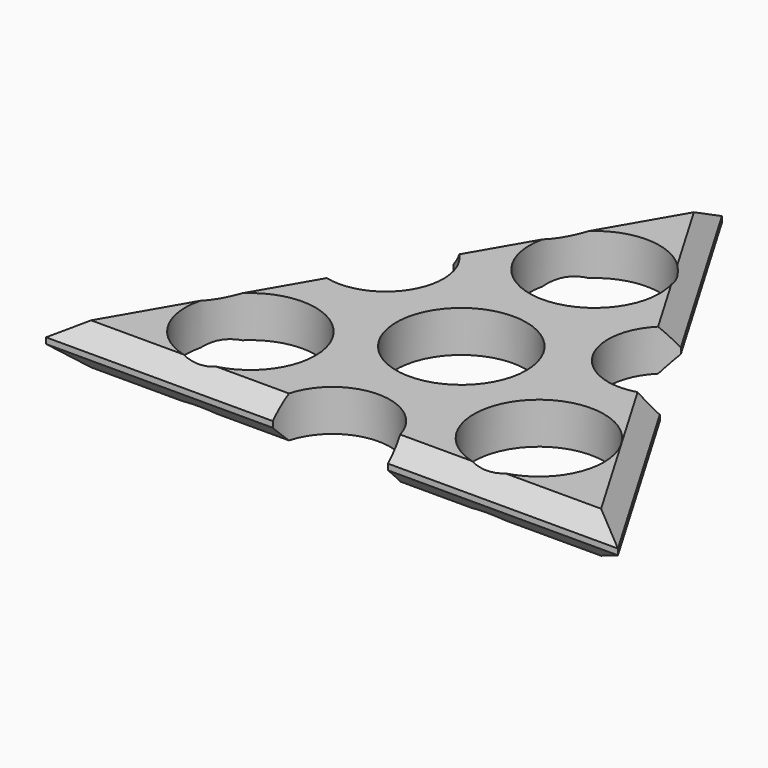
from build123d import *

# Parameters (mm, degrees)
F0_R         = 11
F1_DEPTH     = 7
F2_T1_DEPTH  = 53.4348218988
F2_T3_DEPTH  = 53.3566125342
F2_T5_DEPTH  = 53.6604130231
F2_T7_DEPTH  = 53.7564599562
F2_T9_DEPTH  = 54.3050348939
F2_T11_DEPTH = 54.0874720662
F3_T1_DEPTH  = 53.4348218988
F3_T3_DEPTH  = 53.6604130231
F3_T5_DEPTH  = 53.7564599562
F3_T7_DEPTH  = 54.3050348939
F3_T9_DEPTH  = 54.0874720662
F3_T11_DEPTH = 53.3566125342


# Not quite as in the source:
# - a fillet or chamfer that OpenCascade refuses, or shapes differently, is made with other operations: its cross-section is extruded or revolved along the edge and cut away or added


with BuildPart() as f1:
    # F0 (on Top) → F1 (new body)
    with BuildSketch(Plane.XY):
        with BuildLine():
            Line((19.2151323873, 22.3788071315), (0, 55.077418685))
            Line((0, 55.077418685), (-19.066227053, 22.2013174855))
            ThreePointArc((-19.066227053, 22.2013174855), (-15.2197508504, 8.7138440156), (-28.8366321548, 5.35410246))
            Line((-28.8366321548, 5.35410246), (-48.0160338648, -27.7171470225))
            Line((-48.0160338648, -27.7171470225), (-9.6896718364, -27.7171470225))
            ThreePointArc((-9.6896718364, -27.7171470225), (0.0445471902, -17.5375945189), (9.7787662169, -27.7171470225))
            Line((9.7787662169, -27.7171470225), (48.6537031829, -27.7171470225))
            Line((48.6537031829, -27.7171470225), (29.0682872932, 5.6115802214))
            ThreePointArc((29.0682872932, 5.6115802214), (15.2034219667, 8.7426653076), (19.2151323873, 22.3788071315))
        make_face()
        with Locations((-24.3902284877, -14.0817042541)):
            Circle(F0_R, mode=Mode.SUBTRACT)
        Circle(F0_R, mode=Mode.SUBTRACT)
        with Locations((24.3902285123, -14.0817042399)):
            Circle(F0_R, mode=Mode.SUBTRACT)
        with Locations((0, 28.1634107232)):
            Circle(F0_R, mode=Mode.SUBTRACT)
    extrude(amount=F1_DEPTH)

    # F2: chamfer of 3 on 6 edges, made by hand

    # F2_s2 → F2_t1 (cut)
    with BuildSketch(Plane(origin=(27.7729977796, 47.8892799857, 0), x_dir=(0, 0, 1), z_dir=(-0.5016804508, -0.8650530188, 0))):
        Polygon((4, 27.6312642329), (7, 24.6312642329), (7, 27.6312642329), align=None)
    extrude(amount=F2_T1_DEPTH, mode=Mode.SUBTRACT)

    # F2_s4 → F2_t3 (cut)
    with BuildSketch(Plane(origin=(-0.9341553956, 1.5896629696, 0), x_dir=(0, 0, 1), z_dir=(-0.5066411345, 0.8621570396, 0))):
        Polygon((4, 27.9044858871), (7, 24.9044858871), (7, 27.9044858871), align=None)
    extrude(amount=F2_T3_DEPTH, mode=Mode.SUBTRACT)

    # F2_s6 → F2_t5 (cut)
    with BuildSketch(Plane(origin=(-1.0636343753, -1.8340362392, 0), x_dir=(0, 0, 1), z_dir=(-0.5016804508, -0.8650530188, 0))):
        Polygon((4, 27.6312642329), (7, 24.6312642329), (7, 27.6312642329), align=None)
    extrude(amount=F2_T5_DEPTH, mode=Mode.SUBTRACT)

    # F2_s8 → F2_t7 (cut)
    with BuildSketch(Plane.YZ.offset(-55.7310828287)):
        Polygon((-27.7171470225, 4), (-24.7171470225, 7), (-27.7171470225, 7), align=None)
    extrude(amount=F2_T7_DEPTH, mode=Mode.SUBTRACT)

    # F2_s10 → F2_t9 (cut)
    with BuildSketch(Plane.YZ.offset(2.063717253)):
        Polygon((-27.7171470225, 4), (-24.7171470225, 7), (-27.7171470225, 7), align=None)
    extrude(amount=F2_T9_DEPTH, mode=Mode.SUBTRACT)

    # F2_s12 → F2_t11 (cut)
    with BuildSketch(Plane(origin=(28.5044154, -48.5062911843, 0), x_dir=(0, 0, 1), z_dir=(-0.5066411345, 0.8621570396, 0))):
        Polygon((4, 27.9044858871), (7, 24.9044858871), (7, 27.9044858871), align=None)
    extrude(amount=F2_T11_DEPTH, mode=Mode.SUBTRACT)

    # F3: chamfer of 3 on 6 edges, made by hand

    # F3_s2 → F3_t1 (cut)
    with BuildSketch(Plane(origin=(27.7729977796, 47.8892799857, 0), x_dir=(0, 0, 1), z_dir=(-0.5016804508, -0.8650530188, 0))):
        Polygon((0, 24.6312642329), (3, 27.6312642329), (0, 27.6312642329), align=None)
    extrude(amount=F3_T1_DEPTH, mode=Mode.SUBTRACT)

    # F3_s4 → F3_t3 (cut)
    with BuildSketch(Plane(origin=(-1.0636343753, -1.8340362392, 0), x_dir=(0, 0, 1), z_dir=(-0.5016804508, -0.8650530188, 0))):
        Polygon((0, 24.6312642329), (3, 27.6312642329), (0, 27.6312642329), align=None)
    extrude(amount=F3_T3_DEPTH, mode=Mode.SUBTRACT)

    # F3_s6 → F3_t5 (cut)
    with BuildSketch(Plane.YZ.offset(-55.7310828287)):
        Polygon((-24.7171470225, 0), (-27.7171470225, 3), (-27.7171470225, 0), align=None)
    extrude(amount=F3_T5_DEPTH, mode=Mode.SUBTRACT)

    # F3_s8 → F3_t7 (cut)
    with BuildSketch(Plane.YZ.offset(2.063717253)):
        Polygon((-24.7171470225, 0), (-27.7171470225, 3), (-27.7171470225, 0), align=None)
    extrude(amount=F3_T7_DEPTH, mode=Mode.SUBTRACT)

    # F3_s10 → F3_t9 (cut)
    with BuildSketch(Plane(origin=(28.5044154, -48.5062911843, 0), x_dir=(0, 0, 1), z_dir=(-0.5066411345, 0.8621570396, 0))):
        Polygon((0, 24.9044858871), (3, 27.9044858871), (0, 27.9044858871), align=None)
    extrude(amount=F3_T9_DEPTH, mode=Mode.SUBTRACT)

    # F3_s12 → F3_t11 (cut)
    with BuildSketch(Plane(origin=(-0.9341553956, 1.5896629696, 0), x_dir=(0, 0, 1), z_dir=(-0.5066411345, 0.8621570396, 0))):
        Polygon((0, 24.9044858871), (3, 27.9044858871), (0, 27.9044858871), align=None)
    extrude(amount=F3_T11_DEPTH, mode=Mode.SUBTRACT)


solid = f1.part
